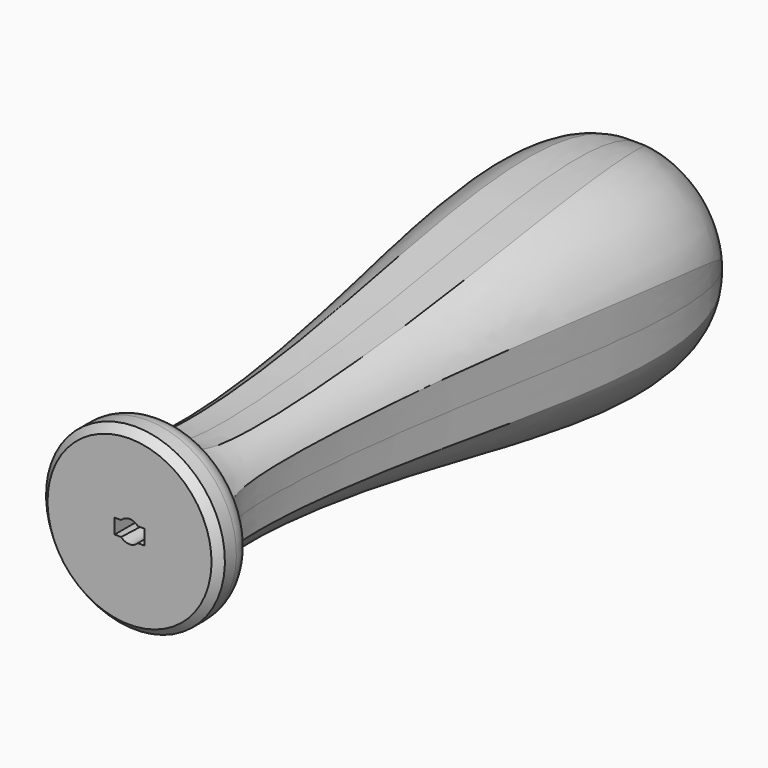
from build123d import *

# Parameters (mm, degrees)
F2_SIZE       = 1
F4_DEPTH      = 5
F4_DEPTH_BACK = 5
F5_COUNT      = 4
F7_R          = 1.5
F8_DEPTH      = 100
F8_DEPTH_BACK = 25
F9_W          = 4
F9_H          = 2
F10_DEPTH     = 25
F10_TAPER     = -1


# Not quite as in the source:
# - the dataset's text gives a spline's control points without its knots; the knots are read off the source's solid


with BuildPart() as f1:
    # F0 (on Right) → F1 (revolve)
    with BuildSketch(Plane.YZ):
        with BuildLine():
            Line((0, 12), (0, 0))
            Line((0, 0), (81.1578258872, 0))
            Line((81.1578258872, 0), (89.6560251713, 0))
            add(Edge.make_bspline(
                [(5.9228962956, 9.1504249722), (6.8900343031, 6.3685388304), (39.5618614962, 7.74400636), (85.7912643516, 19.6263415757), (89.6566016099, 4.5940827585), (89.6560251713, 0)],
                knots=[0, 0, 0, 0, 0.3442049299, 0.770390417, 1, 1, 1, 1], degree=3))
            ThreePointArc((5.9228962956, 9.1504249722), (4.9941231012, 11.1738531363), (2.9266699477, 12))
            Line((2.9266699477, 12), (0, 12))
        make_face()
    revolve(axis=Axis((0, 40.5789129436, 0), (0, -1, 0)))

    # F2
    f2_edges = [f1.edges().sort_by_distance(p)[0] for p in [
        (0, 0, -12),
    ]]
    chamfer(f2_edges, length=F2_SIZE)


with BuildPart() as f4:
    # F3 (on Right) → F4 (new body, two sides)
    with BuildSketch(Plane.YZ) as f4_sk:
        with BuildLine():
            Line((9.9051892757, 31.0736633837), (5.8965189382, 9.1559858993))
            add(Edge.make_bspline(
                [(5.8965189382, 9.1559858993), (5.9472195677, 9.0115264008), (6.0787007332, 8.737855916), (6.4264167356, 8.2752529498), (6.9540357429, 7.8492817721), (7.6695442866, 7.4849318101), (8.477817305, 7.2057885171), (9.3889273865, 6.9862523042), (10.7476798966, 6.7569867165), (12.7180994024, 6.573641292), (15.4916643071, 6.4956271004), (18.6289754692, 6.5476748187), (22.078511792, 6.7198568853), (27.0212738393, 7.0977311992), (32.3663475985, 7.6806858139), (37.8866306932, 8.4350672988), (42.0526870012, 9.0778266944), (46.2117571502, 9.7683310663), (51.7119278945, 10.714634681), (58.4302704603, 11.8739992087), (66.0089075261, 12.9994054756), (72.8627638727, 13.633285281), (77.7556936417, 13.5687704983), (81.0348580655, 13.0706857657), (82.7880556534, 12.5628486358), (83.9981341745, 12.0377737343), (85.0789008782, 11.432460952), (86.1265707678, 10.6022255642), (86.8008379577, 9.8405494507), (87.0694741607, 9.4896582887)],
                knots=[0, 0, 0, 0, 0.0078125, 0.015625, 0.03125, 0.046875, 0.0625, 0.078125, 0.09375, 0.125, 0.15625, 0.1875, 0.21875, 0.25, 0.3125, 0.34375, 0.375, 0.40625, 0.4375, 0.5, 0.5625, 0.625, 0.6875, 0.71875, 0.75, 0.765625, 0.78125, 0.8125, 0.8365570463, 0.8365570463, 0.8365570463, 0.8365570463], degree=3))
            Line((87.0694741607, 9.4896582887), (93.1284055114, 31.0736633837))
            Line((93.1284055114, 31.0736633837), (9.9051892757, 31.0736633837))
        make_face()
    extrude(amount=F4_DEPTH)
    extrude(f4_sk.sketch, amount=-F4_DEPTH_BACK)


with BuildPart() as f5_1:
    # F5: instance of F4
    add(f4.part.rotate(Axis((0, 0, 0), (0, -1, 0)), 1 * 360 / F5_COUNT))


with BuildPart() as f5_2:
    # F5: instance of F4
    add(f4.part.rotate(Axis((0, 0, 0), (0, -1, 0)), 2 * 360 / F5_COUNT))


with BuildPart() as f5_3:
    # F5: instance of F4
    add(f4.part.rotate(Axis((0, 0, 0), (0, -1, 0)), 3 * 360 / F5_COUNT))


with BuildPart() as f1_1:
    add(f1.part)

    # F6: cut F4, F5_1, F5_2, F5_3
    add(f4.part, mode=Mode.SUBTRACT)
    add(f5_1.part, mode=Mode.SUBTRACT)
    add(f5_2.part, mode=Mode.SUBTRACT)
    add(f5_3.part, mode=Mode.SUBTRACT)

    # F7 (on Front) → F8 (cut, two sides)
    with BuildSketch(Plane.XZ) as f8_sk:
        Circle(F7_R)
    extrude(amount=-F8_DEPTH, mode=Mode.SUBTRACT)
    extrude(f8_sk.sketch, amount=F8_DEPTH_BACK, mode=Mode.SUBTRACT)

    # F9 (on Front) → F10 (cut)
    with BuildSketch(Plane.XZ):
        Rectangle(F9_W, F9_H)
    extrude(amount=-F10_DEPTH, taper=F10_TAPER, mode=Mode.SUBTRACT)


solid = f1_1.part
